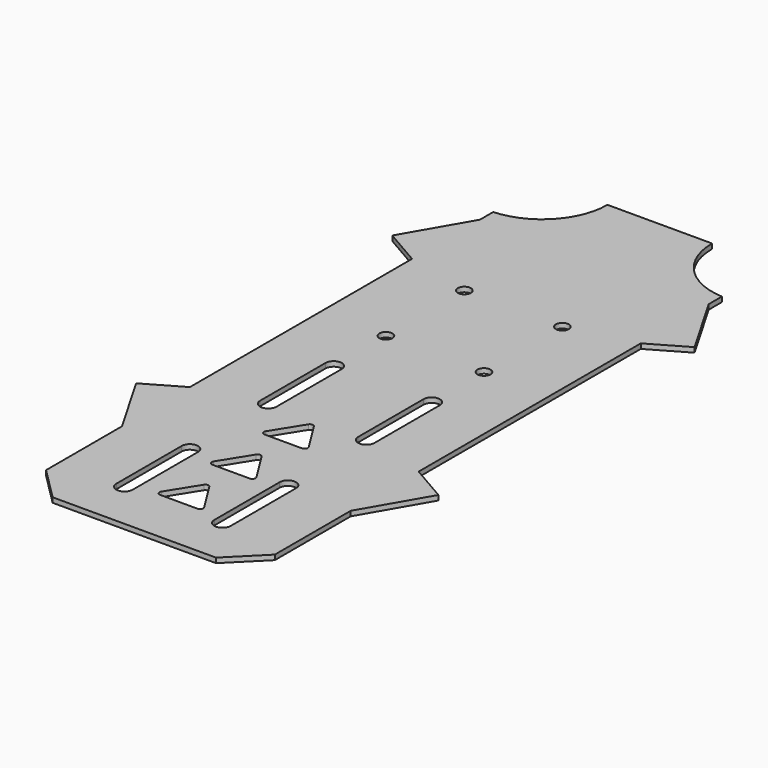
from build123d import *

# Parameters (mm, degrees)
F2_DEPTH = 1.5
F3_R     = 2
F4_DEPTH = 25


# Not quite as in the source:
# - a pattern or mirror of a feature is missing from the dataset's text; its kind, count and spacing are read off the source's solid


with BuildPart() as f2:
    # F1 (on Top) → F2 (new body)
    with BuildSketch(Plane.XY):
        Polygon((-35, -100.5), (35, -100.5), (35, -65.5111069989), (33.25, -64.5007440278), (35, -61.4696551146), (35, -35.4888930011), (35, 49.4888930011), (35, 75.4696551146), (33.25, 78.5007440278), (35, 79.5111069989), (35, 100.5), (-35, 100.5), (-35, 79.5111069989), (-33.25, 78.5007440278), (-35, 75.4696551146), (-35, 49.4888930011), (-35, -35.4888930011), (-35, -61.4696551146), (-33.25, -64.5007440278), (-35, -65.5111069989), align=None)
        Polygon((-46.25, 55.9840835295), (-35, 49.4888930011), (-35, 75.4696551146), align=None)
        Polygon((35, 75.4696551146), (35, 49.4888930011), (46.25, 55.9840835295), align=None)
        Polygon((35, -35.4888930011), (35, -61.4696551146), (46.25, -41.9840835295), align=None)
        Polygon((-46.25, -41.9840835295), (-35, -61.4696551146), (-35, -35.4888930011), align=None)
        Polygon((-35, 79.5111069989), (-35, 75.4696551146), (-33.25, 78.5007440278), align=None)
        Polygon((33.25, 78.5007440278), (35, 75.4696551146), (35, 79.5111069989), align=None)
        Polygon((33.25, -64.5007440278), (35, -65.5111069989), (35, -61.4696551146), align=None)
        Polygon((-35, -61.4696551146), (-35, -65.5111069989), (-33.25, -64.5007440278), align=None)
    extrude(amount=F2_DEPTH)

    # F3 (on face) → F4 (cut)
    with BuildSketch(Plane.XY.offset(1.5)):
        Polygon((-25, -100.5), (-35, -90.5), (-35, -100.5), align=None)
        with BuildLine():
            Line((-12.5, -85.5), (-12.5, -60.5))
            ThreePointArc((-12.5, -60.5), (-15, -58), (-17.5, -60.5))
            Line((-17.5, -60.5), (-17.5, -85.5))
            ThreePointArc((-17.5, -85.5), (-15, -88), (-12.5, -85.5))
        make_face()
        with BuildLine():
            ThreePointArc((-17.5, -30.5), (-15, -33), (-12.5, -30.5))
            Line((-12.5, -30.5), (-12.5, -5.5))
            ThreePointArc((-12.5, -5.5), (-15, -3), (-17.5, -5.5))
            Line((-17.5, -5.5), (-17.5, -30.5))
        make_face()
        with BuildLine():
            Line((17.5, -85.5), (17.5, -60.5))
            ThreePointArc((17.5, -60.5), (15, -58), (12.5, -60.5))
            Line((12.5, -60.5), (12.5, -85.5))
            ThreePointArc((12.5, -85.5), (15, -88), (17.5, -85.5))
        make_face()
        with BuildLine():
            Line((12.5, -5.5), (12.5, -30.5))
            ThreePointArc((12.5, -30.5), (15, -33), (17.5, -30.5))
            Line((17.5, -30.5), (17.5, -5.5))
            ThreePointArc((17.5, -5.5), (15, -3), (12.5, -5.5))
        make_face()
        Polygon((35, -100.5), (35, -90.5), (25, -100.5), align=None)
        with BuildLine():
            ThreePointArc((-6.5437506625, -81.97000106), (-6.5703948397, -82.9847685324), (-5.6957523585, -83.5))
            Line((-5.6957523585, -83.5), (0, -83.5))
            Line((0, -83.5), (5.6957523585, -83.5))
            ThreePointArc((5.6957523585, -83.5), (6.5703948397, -82.9847685324), (6.5437506625, -81.97000106))
            Line((6.5437506625, -81.97000106), (0.847998304, -72.8567972864))
            ThreePointArc((0.847998304, -72.8567972864), (0, -72.3867962264), (-0.847998304, -72.8567972864))
            Line((-0.847998304, -72.8567972864), (-6.5437506625, -81.97000106))
        make_face()
        with BuildLine():
            Line((0, -63.5), (5.6957523585, -63.5))
            ThreePointArc((5.6957523585, -63.5), (6.5703948397, -62.9847685324), (6.5437506625, -61.97000106))
            Line((6.5437506625, -61.97000106), (0.847998304, -52.8567972864))
            ThreePointArc((0.847998304, -52.8567972864), (0, -52.3867962264), (-0.847998304, -52.8567972864))
            Line((-0.847998304, -52.8567972864), (-6.5437506625, -61.97000106))
            ThreePointArc((-6.5437506625, -61.97000106), (-6.5703948397, -62.9847685324), (-5.6957523585, -63.5))
            Line((-5.6957523585, -63.5), (0, -63.5))
        make_face()
        with BuildLine():
            Line((0, -43.5), (5.6957523585, -43.5))
            ThreePointArc((5.6957523585, -43.5), (6.5703948397, -42.9847685324), (6.5437506625, -41.97000106))
            Line((6.5437506625, -41.97000106), (0.847998304, -32.8567972864))
            ThreePointArc((0.847998304, -32.8567972864), (0, -32.3867962264), (-0.847998304, -32.8567972864))
            Line((-0.847998304, -32.8567972864), (-6.5437506625, -41.97000106))
            ThreePointArc((-6.5437506625, -41.97000106), (-6.5703948397, -42.9847685324), (-5.6957523585, -43.5))
            Line((-5.6957523585, -43.5), (0, -43.5))
        make_face()
        with Locations((-15, 14.5)):
            Circle(F3_R)
        with Locations((-15, 44.5)):
            Circle(F3_R)
        with Locations((15, 14.5)):
            Circle(F3_R)
        with Locations((15, 44.5)):
            Circle(F3_R)
        with BuildLine():
            ThreePointArc((56, 100.5), (36, 120.5), (16, 100.5))
            Line((16, 100.5), (35, 100.5))
            Line((35, 100.5), (35, 80.5250156446))
            ThreePointArc((35, 80.5250156446), (49.7840487521, 86.0086232538), (56, 100.5))
        make_face()
        with BuildLine():
            Line((35, 100.5), (16, 100.5))
            ThreePointArc((16, 100.5), (21.5086232538, 86.7159512479), (35, 80.5250156446))
            Line((35, 80.5250156446), (35, 100.5))
        make_face()
    f4 = extrude(amount=-F4_DEPTH, mode=Mode.SUBTRACT)

    # F4_copies: F4 across plane
    add(f4.mirror(Plane(origin=(0, 0, 0), x_dir=(0, 0, -1), z_dir=(-1, 0, 0))), mode=Mode.SUBTRACT)


solid = f2.part
